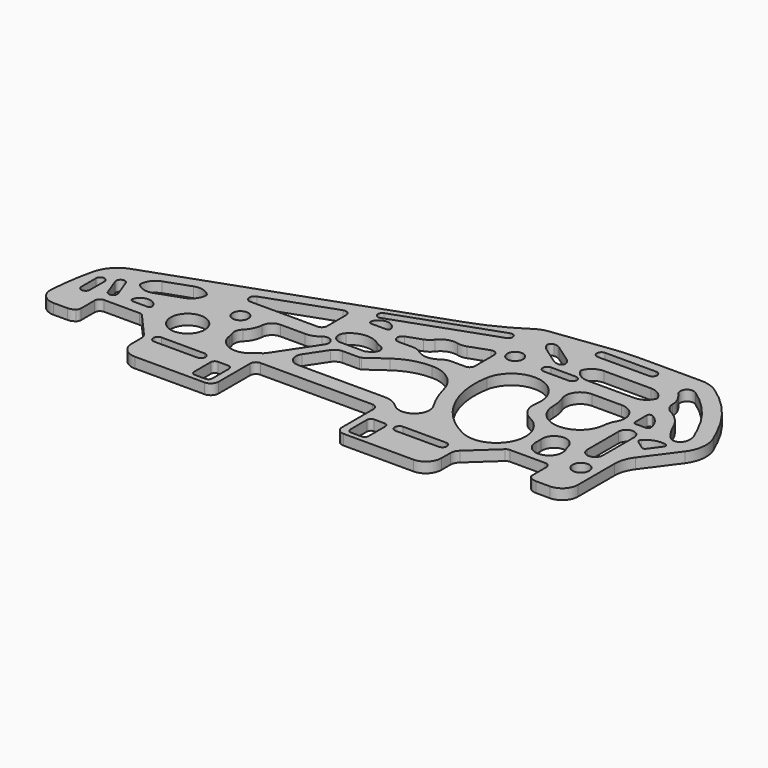
from build123d import *

# Parameters (mm, degrees)
F0_R     = 3.25
F0_R_2   = 1.5
F0_R_3   = 1.6
F1_DEPTH = 2


# Not quite as in the source:
# - ends of sketch curves that miss each other by under 0.0002 mm in the source are joined


with BuildPart() as f1:
    # F0 (on Top) → F1 (new body)
    with BuildSketch(Plane.XY):
        with BuildLine():
            Line((40.512603, 23.481789), (29.131138, 23.481789))
            ThreePointArc((29.131138, 23.481789), (26.3012012992, 23.3918093587), (23.4826968809, 23.1222339314))
            Line((23.4826968809, 23.1222339314), (12.541684, 21.723652))
            ThreePointArc((12.541684, 21.723652), (11.4330846325, 21.4505204175), (10.4153502897, 20.9330165624))
            ThreePointArc((10.4153502897, 20.9330165624), (5.7781096791, 18.2525297039), (0.8502779949, 16.1536050144))
            Line((0.8502779949, 16.1536050144), (-49.030999, -1.599885))
            ThreePointArc((-49.030999, -1.599885), (-51.4858946478, -3.2465293381), (-52.8566147278, -5.8655130647))
            ThreePointArc((-52.8566147278, -5.8655130647), (-53.6653577177, -10.0516682708), (-54.1163267089, -14.2913130185))
            ThreePointArc((-54.1163267089, -14.2913130185), (-53.3100078244, -16.5346622566), (-51.12238, -17.48179))
            Line((-51.12238, -17.48179), (-48.440844, -17.48179))
            ThreePointArc((-48.440844, -17.48179), (-47.7835331419, -17.3706897951), (-47.1992496549, -17.0497324358))
            ThreePointArc((-47.1992496549, -17.0497324358), (-46.9198255904, -16.7011934445), (-46.820047, -16.265761))
            Line((-46.820047, -16.265761), (-46.820047, -12.98179))
            ThreePointArc((-46.820047, -12.98179), (-46.5271537812, -12.2746832188), (-45.820047, -11.98179))
            Line((-45.820047, -11.98179), (-39.020047, -11.98179))
            ThreePointArc((-39.020047, -11.98179), (-38.5805488575, -12.0835465014), (-38.2304943017, -12.3681072345))
            Line((-38.2304943017, -12.3681072345), (-34.218141, -16.914728))
            ThreePointArc((-34.218141, -16.914728), (-33.8469993417, -17.5306785838), (-33.717714, -18.238087))
            Line((-33.717714, -18.238087), (-33.717714, -20.48179))
            ThreePointArc((-33.717714, -20.48179), (-32.8390343436, -22.6031103436), (-30.717714, -23.48179))
            Line((-30.717714, -23.48179), (-17.317714, -23.48179))
            ThreePointArc((-17.317714, -23.48179), (-16.2570538282, -23.0424501718), (-15.817714, -21.98179))
            Line((-15.817714, -21.98179), (-15.817714, -14.40679))
            ThreePointArc((-15.817714, -14.40679), (-15.4955314593, -13.6289725407), (-14.717714, -13.30679))
            Line((-14.717714, -13.30679), (6.782286, -13.30679))
            ThreePointArc((6.782286, -13.30679), (7.5601034593, -13.6289725407), (7.882286, -14.40679))
            Line((7.882286, -14.40679), (7.882286, -21.98179))
            ThreePointArc((7.882286, -21.98179), (8.3216258282, -23.0424501718), (9.382286, -23.48179))
            Line((9.382286, -23.48179), (22.782286, -23.48179))
            ThreePointArc((22.782286, -23.48179), (24.9036063436, -22.6031103436), (25.782286, -20.48179))
            Line((25.782286, -20.48179), (25.782286, -18.355609))
            ThreePointArc((25.782286, -18.355609), (25.9495741205, -17.554879853), (26.4234531668, -16.8881031801))
            Line((26.4234531668, -16.8881031801), (31.405835, -12.274683))
            ThreePointArc((31.405835, -12.274683), (31.7302585676, -12.0579104675), (32.112942, -11.98179))
            Line((32.112942, -11.98179), (38.912942, -11.98179))
            ThreePointArc((38.912942, -11.98179), (39.6200487812, -12.2746832188), (39.912942, -12.98179))
            Line((39.912942, -12.98179), (39.912942, -16.653547))
            ThreePointArc((39.912942, -16.653547), (40.6236606426, -17.2627328355), (41.533739, -17.48179))
            Line((41.533739, -17.48179), (44.195651, -17.48179))
            ThreePointArc((44.195651, -17.48179), (46.3169713436, -16.6031103436), (47.195651, -14.48179))
            Line((47.195651, -14.48179), (47.195651, -5.721689))
            ThreePointArc((47.195651, -5.721689), (47.4967832475, -3.8447483139), (48.369953113, -2.1562100835))
            Line((48.369953113, -2.1562100835), (52.948078, 4.040056))
            ThreePointArc((52.948078, 4.040056), (54.0924062031, 7.0065455742), (53.5602266073, 10.1412438169))
            Line((53.5602266073, 10.1412438169), (52.595339, 12.210453))
            ThreePointArc((52.595339, 12.210453), (48.9319731833, 17.9164636057), (43.8846807292, 22.4445586015))
            ThreePointArc((43.8846807292, 22.4445586015), (42.2766010714, 23.2166221104), (40.512603, 23.481789))
        make_face()
        with BuildLine():
            ThreePointArc((-31.467714, -17.85679), (-32.342714, -16.98179), (-31.467714, -16.10679))
            Line((-31.467714, -16.10679), (-23.217714, -16.10679))
            ThreePointArc((-23.217714, -16.10679), (-22.342714, -16.98179), (-23.217714, -17.85679))
            Line((-23.217714, -17.85679), (-31.467714, -17.85679))
        make_face(mode=Mode.SUBTRACT)
        with BuildLine():
            Line((-17.967714, -22.48179), (-19.967714, -22.48179))
            ThreePointArc((-19.967714, -22.48179), (-20.4980440859, -22.2621200859), (-20.717714, -21.73179))
            Line((-20.717714, -21.73179), (-20.717714, -17.73179))
            ThreePointArc((-20.717714, -17.73179), (-20.4980440859, -17.2014599141), (-19.967714, -16.98179))
            Line((-19.967714, -16.98179), (-17.967714, -16.98179))
            ThreePointArc((-17.967714, -16.98179), (-17.4373839141, -17.2014599141), (-17.217714, -17.73179))
            Line((-17.217714, -17.73179), (-17.217714, -21.73179))
            ThreePointArc((-17.217714, -21.73179), (-17.4373839141, -22.2621200859), (-17.967714, -22.48179))
        make_face(mode=Mode.SUBTRACT)
        with BuildLine():
            ThreePointArc((-51.1775239998, -7.239938), (-50.3525075, -6.4149550002), (-49.5275240002, -7.239971))
            Line((-49.527524, -7.239971), (-49.527595, -10.739971))
            ThreePointArc((-49.5275950002, -10.739971), (-50.3526115, -11.5649549998), (-51.1775949998, -10.739938))
            Line((-51.177595, -10.739938), (-51.177524, -7.239938))
        make_face(mode=Mode.SUBTRACT)
        with BuildLine():
            ThreePointArc((-45.4957372463, -8.9390510929), (-45.9766260929, -10.0020637537), (-47.0396387537, -9.5211749071))
            Line((-47.0396387537, -9.5211749071), (-48.274448, -6.246233))
            ThreePointArc((-48.274448, -6.246233), (-47.79355951, -5.1832204735), (-46.7305467008, -5.6641078872))
            Line((-46.7305467008, -5.6641078872), (-45.4957372463, -8.9390510929))
        make_face(mode=Mode.SUBTRACT)
        with BuildLine():
            Line((-39.36316, -9.633551), (-42.191587, -9.633551))
            ThreePointArc((-42.191587, -9.633551), (-42.5998351591, -9.4222263203), (-42.6629916724, -8.9668847623))
            ThreePointArc((-42.6629916724, -8.9668847623), (-40.777373, -7.633551), (-38.8917547166, -8.9668848998))
            ThreePointArc((-38.8917547166, -8.9668848998), (-38.9549119371, -9.4222264564), (-39.36316, -9.633551))
        make_face(mode=Mode.SUBTRACT)
        with Locations((-31.240863, -10.13869)):
            Circle(F0_R, mode=Mode.SUBTRACT)
        with BuildLine():
            ThreePointArc((-34.9182417778, -0.9247837916), (-34.8118580911, -1.0992111918), (-34.7841267677, -1.3016300162))
            ThreePointArc((-34.7841267677, -1.3016300162), (-35.3872435627, -2.9067375552), (-36.7710009647, -3.9193260992))
            Line((-36.7710009647, -3.9193260992), (-41.481581, -5.595762))
            ThreePointArc((-41.481581, -5.595762), (-43.1939327912, -5.685039278), (-44.6754882694, -4.8218402527))
            ThreePointArc((-44.6754882694, -4.8218402527), (-44.7818719089, -4.6474128082), (-44.8096032323, -4.4449939838))
            ThreePointArc((-44.8096032323, -4.4449939838), (-44.2064864373, -2.8398864448), (-42.8227290353, -1.8272979008))
            Line((-42.8227290353, -1.8272979008), (-38.112149, -0.150862))
            ThreePointArc((-38.112149, -0.150862), (-36.3997972088, -0.061584722), (-34.9182417778, -0.9247837916))
        make_face(mode=Mode.SUBTRACT)
        with BuildLine():
            ThreePointArc((-12.8914672348, -0.8369777084), (-11.1748632273, -0.8897118414), (-10.9642627799, -2.594164146))
            Line((-10.9642627799, -2.594164146), (-15.985231, -10.164332))
            ThreePointArc((-15.985231, -10.164332), (-16.2982291321, -10.5310917453), (-16.6899055583, -10.812285805))
            ThreePointArc((-16.6899055583, -10.812285805), (-17.1780688626, -11.127056177), (-17.6168518029, -11.5076521971))
            ThreePointArc((-17.6168518029, -11.5076521971), (-21.3317967336, -12.3891210944), (-23.788276857, -9.4661931264))
            ThreePointArc((-23.788276857, -9.4661931264), (-23.8810385326, -8.9983473717), (-24.0187982081, -8.541722074))
            ThreePointArc((-24.0187982081, -8.541722074), (-24.0818259305, -7.4169218878), (-23.5269223295, -6.4364986911))
            ThreePointArc((-23.5269223295, -6.4364986911), (-22.5887877044, -5.1230148608), (-22.1744970765, -3.5629829939))
            ThreePointArc((-22.1744970765, -3.5629829939), (-21.5378523692, -2.2521946612), (-20.180775, -1.721324))
            Line((-20.180775, -1.721324), (-15.399991, -1.721324))
            ThreePointArc((-15.399991, -1.721324), (-14.0700699075, -1.493764487), (-12.8914672348, -0.8369777084))
        make_face(mode=Mode.SUBTRACT)
        with Locations((-26.660371, -3.206715)):
            Circle(F0_R_2, mode=Mode.SUBTRACT)
        with BuildLine():
            Line((12.032286, -22.48179), (10.032286, -22.48179))
            ThreePointArc((10.032286, -22.48179), (9.5019559141, -22.2621200859), (9.282286, -21.73179))
            Line((9.282286, -21.73179), (9.282286, -17.73179))
            ThreePointArc((9.282286, -17.73179), (9.5019559141, -17.2014599141), (10.032286, -16.98179))
            Line((10.032286, -16.98179), (12.032286, -16.98179))
            ThreePointArc((12.032286, -16.98179), (12.5626160859, -17.2014599141), (12.782286, -17.73179))
            Line((12.782286, -17.73179), (12.782286, -21.73179))
            ThreePointArc((12.782286, -21.73179), (12.5626160859, -22.2621200859), (12.032286, -22.48179))
        make_face(mode=Mode.SUBTRACT)
        with BuildLine():
            ThreePointArc((14.907286, -17.85679), (14.032286, -16.98179), (14.907286, -16.10679))
            Line((14.907286, -16.10679), (23.157286, -16.10679))
            ThreePointArc((23.157286, -16.10679), (24.032286, -16.98179), (23.157286, -17.85679))
            Line((23.157286, -17.85679), (14.907286, -17.85679))
        make_face(mode=Mode.SUBTRACT)
        with BuildLine():
            ThreePointArc((-9.157645555, -3.4887006319), (-8.436726467, -2.8319315045), (-7.490927, -2.594164))
            Line((-7.490927, -2.594164), (-4.233575, -2.594164))
            ThreePointArc((-4.233575, -2.594164), (-4.0820976551, -2.5706664806), (-3.9448576776, -2.5023824559))
            Line((-3.9448576776, -2.5023824559), (-0.485977, -0.05605))
            ThreePointArc((-0.485977, -0.05605), (2.5782632754, 1.4685670305), (5.960389, 1.99321))
            ThreePointArc((5.960389, 1.99321), (9.8546591217, 0.6492077073), (12.091018298, -2.8106159266))
            ThreePointArc((12.091018298, -2.8106159266), (12.9614193732, -5.4513862217), (14.2260258996, -7.9276810614))
            ThreePointArc((14.2260258996, -7.9276810614), (13.5437578661, -11.7361370382), (9.6814241094, -11.5076518906))
            ThreePointArc((9.6814241094, -11.5076518906), (8.3512880727, -10.6188839167), (6.782286, -10.30679))
            Line((6.782286, -10.30679), (-9.953353, -10.30679))
            ThreePointArc((-9.953353, -10.30679), (-11.7155856925, -9.2525890999), (-11.6200710944, -7.2013259374))
            Line((-11.6200710944, -7.2013259374), (-9.157645555, -3.4887006319))
        make_face(mode=Mode.SUBTRACT)
        with BuildLine():
            ThreePointArc((14.7951546308, 4.1402980651), (21.2825079796, 8.6827913843), (25.8250013994, 2.1954381059))
            ThreePointArc((25.8250013994, 2.1954381059), (26.2064100519, -0.2826091703), (28.0175412021, -2.0163895666))
            ThreePointArc((28.0175412021, -2.0163895666), (30.7262024985, -9.4583754993), (23.2842162815, -12.1670363963))
            ThreePointArc((23.2842162815, -12.1670363963), (16.2718885147, -5.4541932436), (14.7951546308, 4.1402980651))
        make_face(mode=Mode.SUBTRACT)
        with BuildLine():
            ThreePointArc((38.5786255222, -6.581078228), (36.7333598097, -10.2510273466), (33.6375187116, -7.5511569834))
            ThreePointArc((33.6375187116, -7.5511569834), (33.6496094111, -6.9593203609), (33.6179037154, -6.368209935))
            ThreePointArc((33.6179037154, -6.368209935), (35.5921267196, -3.8339317819), (38.2510784783, -5.6367351181))
            ThreePointArc((38.2510784783, -5.6367351181), (38.3885508135, -6.1180292822), (38.5786255222, -6.581078228))
        make_face(mode=Mode.SUBTRACT)
        with Locations((44.077012, -9.856887)):
            Circle(F0_R_3, mode=Mode.SUBTRACT)
        with BuildLine():
            Line((41.14007, -4.643382), (41.14007, 2.856618))
            ThreePointArc((41.14007, 2.856618), (42.64007, 4.356618), (44.14007, 2.856618))
            Line((44.14007, 2.856618), (44.14007, -4.643382))
            ThreePointArc((44.14007, -4.643382), (42.64007, -6.143382), (41.14007, -4.643382))
        make_face(mode=Mode.SUBTRACT)
        with BuildLine():
            ThreePointArc((-14.399992, 2.278676), (-14.6928852188, 1.5715692188), (-15.399992, 1.278676))
            Line((-15.399992, 1.278676), (-28.302898, 1.278676))
            ThreePointArc((-28.302898, 1.278676), (-29.2883186889, 2.108540566), (-28.6382079531, 3.2207838682))
            Line((-28.6382079531, 3.2207838682), (-15.735302, 7.813121))
            ThreePointArc((-15.735302, 7.813121), (-14.8234982676, 7.6881145705), (-14.399992, 6.871013))
            Line((-14.399992, 6.871013), (-14.399992, 2.278676))
        make_face(mode=Mode.SUBTRACT)
        with BuildLine():
            ThreePointArc((-10.7614843369, 2.2449993265), (-8.0739443754, 3.5275248045), (-5.2011879423, 2.7432970804))
            ThreePointArc((-5.2011879423, 2.7432970804), (-4.6693197037, 2.4211660931), (-4.0939577701, 2.1853467148))
            ThreePointArc((-4.0939577701, 2.1853467148), (-3.2783121321, 1.2285040194), (-3.7696761681, 0.0711852377))
            Line((-3.7696761681, 0.0711852377), (-4.580645, -0.502382))
            ThreePointArc((-4.580645, -0.502382), (-4.717885266, -0.5706663569), (-4.869363, -0.594164))
            Line((-4.869363, -0.594164), (-9.559223, -0.594164))
            ThreePointArc((-9.559223, -0.594164), (-11.1008357119, 0.4271645953), (-10.7614843369, 2.2449993265))
        make_face(mode=Mode.SUBTRACT)
        with BuildLine():
            Line((-6.881633, 7.035401), (-9.71006, 7.035401))
            ThreePointArc((-9.71006, 7.035401), (-10.1183080629, 7.2467255436), (-10.1814647835, 7.7020669235))
            ThreePointArc((-10.1814647835, 7.7020669235), (-8.2958468333, 9.035401), (-6.4102286055, 7.7020667859))
            ThreePointArc((-6.4102286055, 7.7020667859), (-6.4733849371, 7.2467255436), (-6.881633, 7.035401))
        make_face(mode=Mode.SUBTRACT)
        with BuildLine():
            Line((9.03337, 16.067494), (-9.808786, 9.36129))
            ThreePointArc((-9.808786, 9.36129), (-10.8626559011, 9.8618980352), (-10.3620479648, 10.9157679011))
            Line((-10.3620479648, 10.9157679011), (8.480108, 17.621972))
            ThreePointArc((8.480108, 17.621972), (9.5339779011, 17.1213639648), (9.03337, 16.067494))
        make_face(mode=Mode.SUBTRACT)
        with BuildLine():
            Line((10.033684, 4.99321), (7.332231, 4.99321))
            ThreePointArc((7.332231, 4.99321), (6.3835477019, 4.8392598942), (5.532231, 4.39321))
            ThreePointArc((5.532231, 4.39321), (3.582231, 3.74321), (1.632231, 4.39321))
            ThreePointArc((1.632231, 4.39321), (0.7809142981, 4.8392598942), (-0.167769, 4.99321))
            Line((-0.167769, 4.99321), (-2.869223, 4.99321))
            ThreePointArc((-2.869223, 4.99321), (-3.8546436889, 5.823074566), (-3.2045329531, 6.9353178682))
            Line((-3.2045329531, 6.9353178682), (-0.399099, 7.933814))
            ThreePointArc((-0.399099, 7.933814), (0.3694756464, 8.3412254142), (0.9888554494, 8.9520116606))
            ThreePointArc((0.9888554494, 8.9520116606), (2.4924720644, 10.0550600065), (4.3548788626, 10.1500304384))
            ThreePointArc((4.3548788626, 10.1500304384), (5.2208740922, 10.0679118184), (6.0740238593, 10.2376953954))
            Line((6.0740238593, 10.2376953954), (9.698373, 11.527655))
            ThreePointArc((9.698373, 11.527655), (10.6101773475, 11.4026488421), (11.033684, 10.585547))
            Line((11.033684, 10.585547), (11.033684, 5.99321))
            ThreePointArc((11.033684, 5.99321), (10.7407907812, 5.2861032188), (10.033684, 4.99321))
        make_face(mode=Mode.SUBTRACT)
        with BuildLine():
            ThreePointArc((27.7891688027, 6.0074469251), (28.1067686801, 8.6291364327), (30.445019, 9.856618))
            Line((30.445019, 9.856618), (36.14007, 9.856618))
            ThreePointArc((36.14007, 9.856618), (38.8274594814, 8.2886225969), (38.7847707398, 5.1775371566))
            ThreePointArc((38.7847707398, 5.1775371566), (38.3536543941, 4.2265182412), (38.1533253565, 3.2017419726))
            ThreePointArc((38.1533253565, 3.2017419726), (35.2828977993, -0.9670181189), (30.2396183016, -0.5389475693))
            ThreePointArc((30.2396183016, -0.5389475693), (28.8213440066, 1.0783936909), (28.310078, 3.167868))
            ThreePointArc((28.310078, 3.167868), (28.1787730258, 4.6113494133), (27.7891688027, 6.0074469251))
        make_face(mode=Mode.SUBTRACT)
        with BuildLine():
            ThreePointArc((45.4988999736, 2.8491100258), (47.1838932345, 3.8987751854), (49.1633500895, 4.0496055395))
            ThreePointArc((49.1633500895, 4.0496055395), (49.5448805923, 3.744125237), (49.4836138442, 3.2592231151))
            Line((49.4836138442, 3.2592231151), (47.839895, 1.034618))
            ThreePointArc((47.839895, 1.034618), (47.5120087188, 0.8372927539), (47.1406281151, 0.9296131558))
            Line((47.1406281151, 0.9296131558), (45.559631, 2.097782))
            ThreePointArc((45.559631, 2.097782), (45.358387471, 2.4596336496), (45.4988999736, 2.8491100258))
        make_face(mode=Mode.SUBTRACT)
        with BuildLine():
            Line((43.60582, 6.356618), (41.64007, 6.356618))
            ThreePointArc((41.64007, 6.356618), (41.2865166094, 6.5030646094), (41.14007, 6.856618))
            Line((41.14007, 6.856618), (41.14007, 9.622605))
            ThreePointArc((41.14007, 9.622605), (41.3789535753, 10.049006469), (41.8673428511, 10.0679667082))
            ThreePointArc((41.8673428511, 10.0679667082), (43.369732145, 8.7703431336), (44.1011495134, 6.9248000707))
            ThreePointArc((44.1011495134, 6.9248000707), (43.982709259, 6.5280537194), (43.60582, 6.356618))
        make_face(mode=Mode.SUBTRACT)
        with Locations((13.783684, 12.215472)):
            Circle(F0_R_2, mode=Mode.SUBTRACT)
        with BuildLine():
            ThreePointArc((20.180271, 11.089047), (19.330271, 11.939047), (20.180271, 12.789047))
            Line((20.180271, 12.789047), (24.980271, 12.789047))
            ThreePointArc((24.980271, 12.789047), (25.830271, 11.939047), (24.980271, 11.089047))
            Line((24.980271, 11.089047), (20.180271, 11.089047))
        make_face(mode=Mode.SUBTRACT)
        with BuildLine():
            ThreePointArc((15.8743839633, 18.9664858493), (16.5207733861, 18.8883098411), (17.1077989997, 18.6066509996))
            Line((17.1077989997, 18.6066509996), (20.384407, 16.312345))
            ThreePointArc((20.384407, 16.312345), (20.8498541669, 15.8570543988), (21.1443936963, 15.2763849041))
            ThreePointArc((21.1443936963, 15.2763849041), (21.0449247067, 14.6290707141), (20.470669016, 14.3142056285))
            ThreePointArc((20.470669016, 14.3142056285), (19.8242795932, 14.3923821649), (19.2372540003, 14.6740410004))
            Line((19.2372540003, 14.6740410004), (15.960646, 16.968347))
            ThreePointArc((15.960646, 16.968347), (15.4951988331, 17.4236376012), (15.2006593037, 18.0043070959))
            ThreePointArc((15.2006593037, 18.0043070959), (15.3001285667, 18.6516206764), (15.8743839633, 18.9664858493))
        make_face(mode=Mode.SUBTRACT)
        with BuildLine():
            Line((36.14007, 12.856618), (27.14007, 12.856618))
            ThreePointArc((27.14007, 12.856618), (25.4969023973, 13.3466378747), (24.3905246497, 14.6566178471))
            ThreePointArc((24.3905246497, 14.6566178471), (24.348783, 14.856618), (24.3905253616, 15.0566178422))
            ThreePointArc((24.3905253616, 15.0566178422), (25.4969023973, 16.3665981253), (27.14007, 16.856618))
            Line((27.14007, 16.856618), (36.14007, 16.856618))
            ThreePointArc((36.14007, 16.856618), (37.7832377701, 16.3665980157), (38.8896155103, 15.0566177863))
            ThreePointArc((38.8896155103, 15.0566177863), (38.931358, 14.856618), (38.8896156384, 14.6566181578))
            ThreePointArc((38.8896156384, 14.6566181578), (37.7832377701, 13.3466379843), (36.14007, 12.856618))
        make_face(mode=Mode.SUBTRACT)
        with BuildLine():
            ThreePointArc((50.9567886241, 6.6226147836), (49.8994765997, 5.6868290935), (48.5507912462, 6.104742233))
            ThreePointArc((48.5507912462, 6.104742233), (47.4304590943, 7.5260415419), (46.583603485, 9.1254387843))
            ThreePointArc((46.583603485, 9.1254387843), (45.227903185, 11.2301541088), (43.2309799895, 12.7401369795))
            ThreePointArc((43.2309799895, 12.7401369795), (42.2826874439, 13.6171181596), (41.9313571559, 14.8600670002))
            ThreePointArc((41.9313571559, 14.8600670002), (41.857177348, 15.5733897873), (41.6391609886, 16.256617995))
            ThreePointArc((41.6391609886, 16.256617995), (41.1458745936, 17.1644753686), (40.5041472465, 17.9742422891))
            ThreePointArc((40.5041472465, 17.9742422891), (40.4596540023, 19.7284376841), (42.198641666, 19.9631735085))
            ThreePointArc((42.198641666, 19.9631735085), (46.6474410618, 15.9720066157), (49.8764154209, 10.94259773))
            Line((49.8764154209, 10.94259773), (50.841304, 8.873389))
            ThreePointArc((50.841304, 8.873389), (51.1184388669, 7.7592586445), (50.9567886241, 6.6226147836))
        make_face(mode=Mode.SUBTRACT)
        with BuildLine():
            Line((33.382697, 19.821789), (23.582697, 19.821789))
            ThreePointArc((23.582697, 19.821789), (22.707697, 20.696789), (23.582697, 21.571789))
            Line((23.582697, 21.571789), (33.382697, 21.571789))
            ThreePointArc((33.382697, 21.571789), (34.257697, 20.696789), (33.382697, 19.821789))
        make_face(mode=Mode.SUBTRACT)
    extrude(amount=F1_DEPTH)


solid = f1.part
